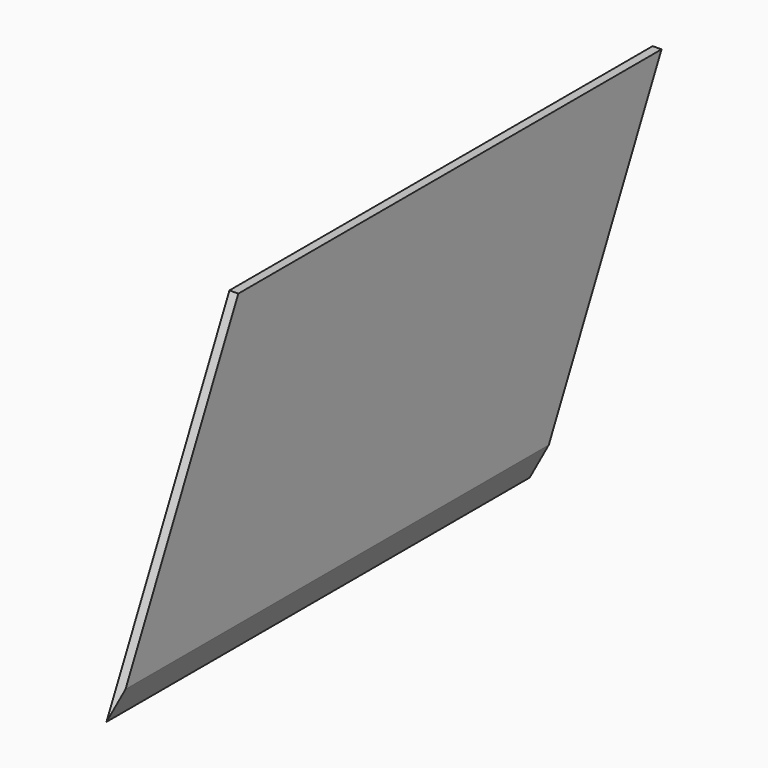
from build123d import *

# Parameters (mm, degrees)
F1_DEPTH = 0.5
F2_SIZE2 = 1.49999
F2_SIZE  = 0.49999


# Not quite as in the source:
# - a fillet or chamfer is up to 0.001 mm smaller than in the source, because OpenCascade refuses the exact size


with BuildPart() as f1:
    # F0 (on Right) → F1 (new body)
    with BuildSketch(Plane.YZ):
        Polygon((15, 0), (-15, 0), (-23.7177978871, -18), (6.2822021129, -18), align=None)
    extrude(amount=F1_DEPTH)

    # F2 (size 0.5 and 1.5 in the source; OpenCascade refuses exactly that, so slightly less here)
    f2_edges = [f1.edges().sort_by_distance(p)[0] for p in [
        (0.5, -8.717798, -18),
    ]]
    f2_side = f1.faces().sort_by_distance((0.25, -8.717798, -18))[0]
    chamfer(f2_edges, length=F2_SIZE, length2=F2_SIZE2, reference=f2_side)


solid = f1.part
